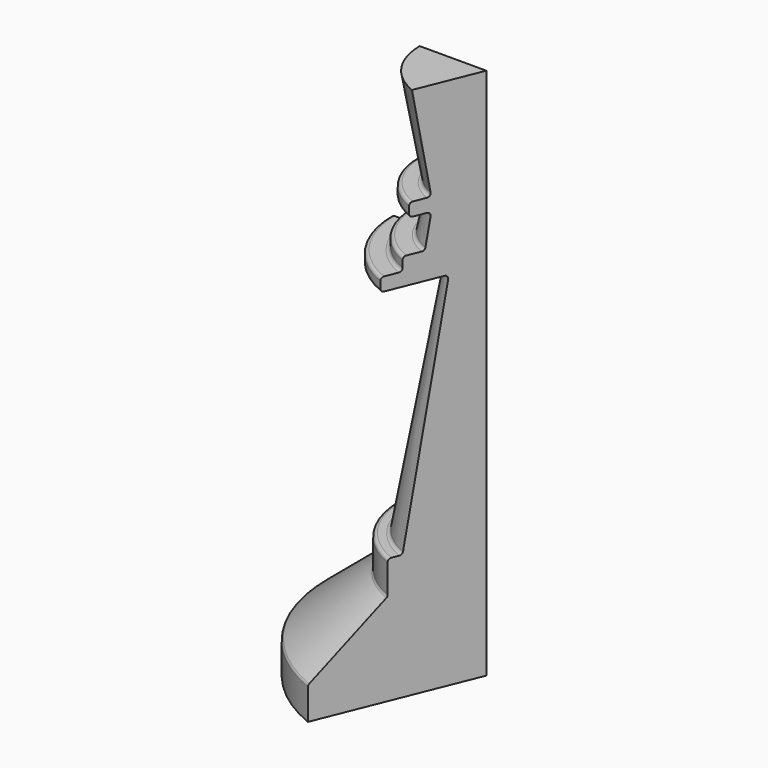
from build123d import *

# Parameters (mm, degrees)
F1_ANGLE = 68


# Not quite as in the source:
# - a feature of the source that left no trace in its solid (it failed there, or was rolled back) is left out


with BuildPart() as f1:
    # F0 (on Front) → F1 (revolve)
    with BuildSketch(Plane.XZ):
        with BuildLine():
            Line((-15.24, 0), (0, 0))
            Line((0, 0), (0, 50.8))
            Line((0, 50.8), (-6.35, 50.8))
            Line((-6.35, 50.8), (-4.7617064118, 41.792339449))
            ThreePointArc((-4.7617064118, 41.792339449), (-4.8311637627, 41.5331210865), (-5.0743828734, 41.4197061526))
            Line((-5.0743828734, 41.4197061526), (-6.2835011077, 41.4197061526))
            ThreePointArc((-6.2835011077, 41.4197061526), (-6.5080075107, 41.3267125556), (-6.6010011077, 41.1022061526))
            Line((-6.6010011077, 41.1022061526), (-6.6010011077, 40.4672061526))
            ThreePointArc((-6.6010011077, 40.4672061526), (-6.5080075107, 40.2426997495), (-6.2835011077, 40.1497061526))
            Line((-6.2835011077, 40.1497061526), (-5.0743828734, 40.1497061526))
            ThreePointArc((-5.0743828734, 40.1497061526), (-4.8311637627, 40.0362912186), (-4.7617064118, 39.7770728561))
            Line((-4.7617064118, 39.7770728561), (-5.2010717431, 37.2853082403))
            ThreePointArc((-5.2010717431, 37.2853082403), (-5.3096631386, 37.0972224261), (-5.5137482047, 37.0229415367))
            Line((-5.5137482047, 37.0229415367), (-6.8348340718, 37.0229415367))
            ThreePointArc((-6.8348340718, 37.0229415367), (-7.0593404748, 36.9299479398), (-7.1523340718, 36.7054415367))
            Line((-7.1523340718, 36.7054415367), (-7.1523340718, 36.0704415367))
            ThreePointArc((-7.1523340718, 36.0704415367), (-7.2453276688, 35.8459351337), (-7.4698340718, 35.7529415367))
            Line((-7.4698340718, 35.7529415367), (-8.7398340718, 35.7529415367))
            ThreePointArc((-8.7398340718, 35.7529415367), (-8.9643404748, 35.6599479398), (-9.0573340718, 35.4354415367))
            Line((-9.0573340718, 35.4354415367), (-9.0573340718, 34.8004415367))
            ThreePointArc((-9.0573340718, 34.8004415367), (-8.9643404748, 34.5759351337), (-8.7398340718, 34.4829415367))
            Line((-8.7398340718, 34.4829415367), (-3.5686493249, 34.4829415367))
            ThreePointArc((-3.5686493249, 34.4829415367), (-3.3254302142, 34.3695266028), (-3.2559728633, 34.1103082403))
            Line((-3.2559728633, 34.1103082403), (-7.113602572, 12.2326030065))
            ThreePointArc((-7.113602572, 12.2326030065), (-7.2221939675, 12.0445171922), (-7.4262790336, 11.9702363029))
            Line((-7.4262790336, 11.9702363029), (-8.1123649007, 11.9702363029))
            ThreePointArc((-8.1123649007, 11.9702363029), (-8.3368713037, 11.8772427059), (-8.4298649007, 11.6527363029))
            Line((-8.4298649007, 11.6527363029), (-8.4298649007, 8.9432889844))
            ThreePointArc((-8.4298649007, 8.9432889844), (-8.4596121783, 8.8091076862), (-8.5432798346, 8.7000698737))
            Line((-8.5432798346, 8.7000698737), (-15.1265850661, 3.176020882))
            ThreePointArc((-15.1265850661, 3.176020882), (-15.2102527224, 3.0669830694), (-15.24, 2.9328017713))
            Line((-15.24, 2.9328017713), (-15.24, 0))
        make_face()
    revolve(axis=Axis((0, 0, 25.4), (0, 0, 1)), revolution_arc=F1_ANGLE)


solid = f1.part
